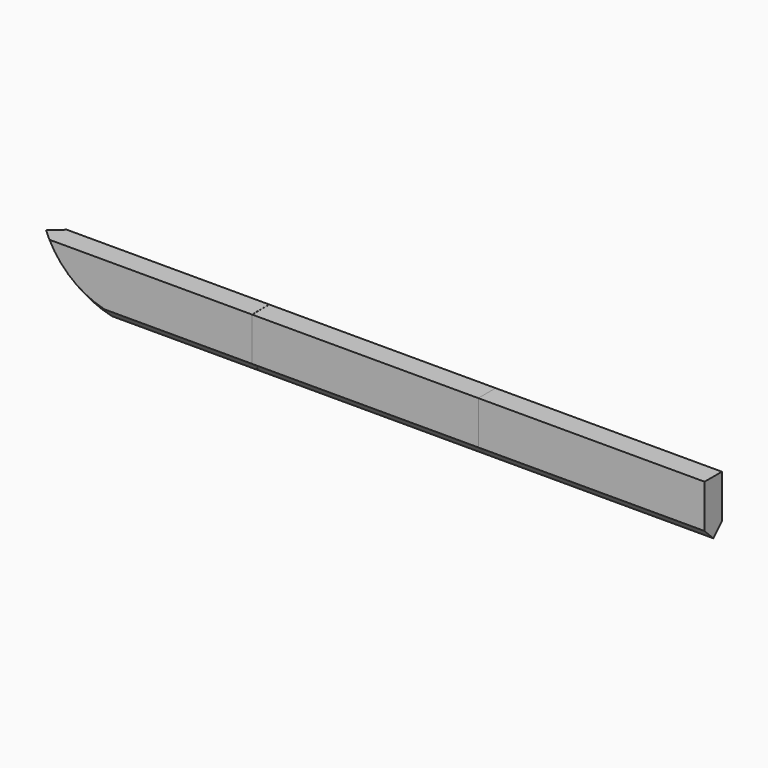
from build123d import *

# Parameters (mm, degrees)
F0_W          = 53
F0_H          = 15.24
F1_DEPTH      = 2.54
F1_DEPTH_BACK = 2.54
F3_DEPTH      = 2.54
F3_DEPTH_BACK = 2.54
F4_W          = 53
F4_H          = 15.24
F5_DEPTH      = 2.54
F5_DEPTH_BACK = 2.54
F6_T1_DEPTH   = 61.2405111475
F6_2_T1_DEPTH = 79.1282991577
F6_3_T1_DEPTH = 79.1282991577
F7_T2_ANGLE   = 87.5032062874
F7_T4_ANGLE   = 87.5032062874


# Not quite as in the source:
# - a fillet or chamfer that OpenCascade refuses, or shapes differently, is made with other operations: its cross-section is extruded or revolved along the edge and cut away or added


with BuildPart() as f1:
    # F0 (on Front) → F1 (new body, two sides)
    with BuildSketch(Plane.XZ) as f1_sk:
        Rectangle(F0_W, F0_H)
    extrude(amount=F1_DEPTH)
    extrude(f1_sk.sketch, amount=-F1_DEPTH_BACK)

    # F6#2: chamfer of 5.08 on 2 edges, made by hand

    # F6_2_s2 → F6_2_t1 (cut)
    with BuildSketch(Plane.YZ.offset(-39.5641495789)):
        Polygon((2.54, -7.62), (-2.54, -2.54), (-2.54, -7.62), align=None)
        Polygon((-2.54, -7.62), (2.54, -2.54), (2.54, -7.62), align=None)
    extrude(amount=F6_2_T1_DEPTH, mode=Mode.SUBTRACT)


with BuildPart() as f3:
    # F2 (on Front) → F3 (new body, two sides)
    with BuildSketch(Plane.XZ) as f3_sk:
        with BuildLine():
            Line((-61.6335310042, -7.62), (-26.5213190144, -7.62))
            Line((-26.5213190144, -7.62), (-26.5213190144, 7.62))
            Line((-26.5213190144, 7.62), (-79.2149826884, 7.62))
            Line((-79.2149826884, 7.62), (-79.2149826884, 6.8744295258))
            ThreePointArc((-79.2149826884, 6.8744295258), (-72.179765207, -2.5021815938), (-61.6335310042, -7.62))
        make_face()
    extrude(amount=F3_DEPTH)
    extrude(f3_sk.sketch, amount=-F3_DEPTH_BACK)

    # F6: chamfer of 5.08 on 2 edges, made by hand

    # F6_s2 → F6_t1 (cut)
    with BuildSketch(Plane.YZ.offset(-74.6976805831)):
        Polygon((2.54, -7.62), (-2.54, -2.54), (-2.54, -7.62), align=None)
        Polygon((-2.54, -7.62), (2.54, -2.54), (2.54, -7.62), align=None)
    extrude(amount=F6_T1_DEPTH, mode=Mode.SUBTRACT)

    # F7: chamfer of 5.08 on 2 edges, made by hand

    # F7_s1 → F7_t2 (revolve, cut)
    with BuildSketch(Plane(origin=(1.1745778192, 0, 9.8467873874), x_dir=(0, 1, 0), z_dir=(0.118445679, 0, 0.9929605335))):
        Polygon((2.54, 82.8215486164), (-2.54, 77.7415486164), (-2.54, 82.8215486164), align=None)
    revolve(axis=Axis((-56.3427767118, -2.54, 16.7077671356), (0, -1, 0)), revolution_arc=F7_T2_ANGLE, mode=Mode.SUBTRACT)

    # F7_s3 → F7_t4 (revolve, cut)
    with BuildSketch(Plane(origin=(1.1745778192, 0, 9.8467873874), x_dir=(0, 1, 0), z_dir=(0.118445679, 0, 0.9929605335))):
        Polygon((-2.54, 82.8215486164), (2.54, 77.7415486164), (2.54, 82.8215486164), align=None)
    revolve(axis=Axis((-56.3427767118, 2.54, 16.7077671356), (0, -1, 0)), revolution_arc=F7_T4_ANGLE, mode=Mode.SUBTRACT)


with BuildPart() as f5:
    # F4 (on Front) → F5 (new body, two sides)
    with BuildSketch(Plane.XZ) as f5_sk:
        with Locations((52.9905296862, 0)):
            Rectangle(F4_W, F4_H)
    extrude(amount=F5_DEPTH)
    extrude(f5_sk.sketch, amount=-F5_DEPTH_BACK)

    # F6#3: chamfer of 5.08 on 2 edges, made by hand

    # F6_3_s2 → F6_3_t1 (cut)
    with BuildSketch(Plane.YZ.offset(13.4263801073)):
        Polygon((-2.54, -7.62), (2.54, -2.54), (2.54, -7.62), align=None)
        Polygon((2.54, -7.62), (-2.54, -2.54), (-2.54, -7.62), align=None)
    extrude(amount=F6_3_T1_DEPTH, mode=Mode.SUBTRACT)


solid = Compound([f1.part, f3.part, f5.part])
